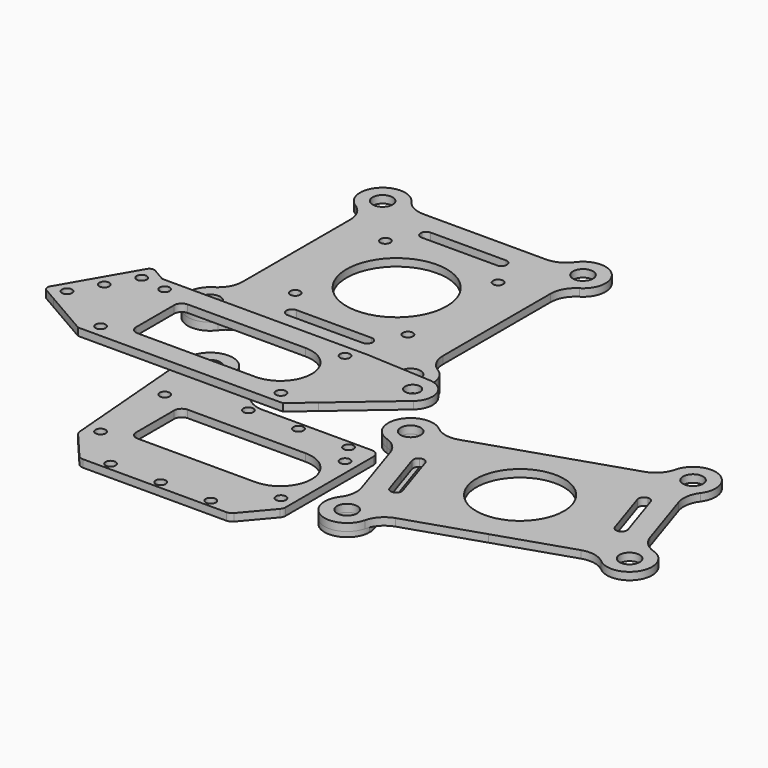
from build123d import *

# Parameters (mm, degrees)
F0_R      = 1
F0_W      = 30
F0_H      = 6.5
F0_R_2    = 2
F1_DEPTH  = 1.5
F3_R      = 2
F4_DEPTH  = 1.5
F5_R      = 5
F5_2_R    = 5
F5_3_R    = 5
F6_R      = 1.5
F7_DEPTH  = 0.5
F8_R      = 8.75
F8_R_2    = 2
F9_DEPTH  = 1.5
F10_R     = 2
F10_R_2   = 1
F10_R_3   = 10
F11_DEPTH = 1.5
F12_R     = 5
F12_2_R   = 5
F14_R     = 1
F14_R_2   = 2
F15_DEPTH = 1.5
F16_R     = 2
F17_DEPTH = 1.5
F18_R     = 1
F19_DEPTH = 1.5
F20_R     = 2
F20_R_2   = 1.5
F21_DEPTH = 1.5


with BuildPart() as f1:
    # F0 (on Top) → F1 (new body)
    with BuildSketch(Plane.XY):
        with BuildLine():
            Line((-32, -10.5), (-32, 10.5))
            Line((-32, 10.5), (9, 10.5))
            Line((9, 10.5), (9, 13.5))
            Line((9, 13.5), (-15.9210526316, 13.5))
            Line((-15.9210526316, 13.5), (-25.5, 20))
            ThreePointArc((-25.5, 20), (-29.8149179926, 15.5038077609), (-34.4847754002, 19.6301492066))
            Line((-34.4847754002, 19.6301492066), (-32, -10.5))
        make_face()
        with Locations((-16, 12)):
            Circle(F0_R, mode=Mode.SUBTRACT)
        with Locations((-6, 12)):
            Circle(F0_R, mode=Mode.SUBTRACT)
        with Locations((4, 12)):
            Circle(F0_R, mode=Mode.SUBTRACT)
        Polygon((9, 10.5), (-32, 10.5), (-32, -10.5), (-26.5, -10.5), (3.5, -10.5), (9, -10.5), align=None)
        with Locations((-29.5, -8)):
            Circle(F0_R, mode=Mode.SUBTRACT)
        with BuildLine():
            ThreePointArc((0, 6.25), (6.25, 0), (0, -6.25))
            Line((0, -6.25), (-23.5, -6.25))
            ThreePointArc((-23.5, -6.25), (-24.5606601718, -5.8106601718), (-25, -4.75))
            Line((-25, -4.75), (-25, 0))
            Line((-25, 0), (-25, 4.75))
            ThreePointArc((-25, 4.75), (-24.5606601718, 5.8106601718), (-23.5, 6.25))
            Line((-23.5, 6.25), (0, 6.25))
        make_face(mode=Mode.SUBTRACT)
        with Locations((6.5, -8)):
            Circle(F0_R, mode=Mode.SUBTRACT)
        with Locations((-29.5, 8)):
            Circle(F0_R, mode=Mode.SUBTRACT)
        with Locations((6.5, 8)):
            Circle(F0_R, mode=Mode.SUBTRACT)
        Polygon((-26.5, -10.5), (-32, -10.5), (-26.5, -17), align=None)
        Polygon((3.5, -17), (9, -10.5), (3.5, -10.5), align=None)
        with Locations((-11.5, -13.75)):
            Rectangle(F0_W, F0_H)
        with Locations((-21.5, -15.5)):
            Circle(F0_R, mode=Mode.SUBTRACT)
        with Locations((-11.5, -15.5)):
            Circle(F0_R, mode=Mode.SUBTRACT)
        with Locations((-1.5, -15.5)):
            Circle(F0_R, mode=Mode.SUBTRACT)
        with BuildLine():
            ThreePointArc((-25.5, 20), (-30.1850820074, 24.4961922391), (-34.4847754002, 19.6301492066))
            ThreePointArc((-34.4847754002, 19.6301492066), (-29.8149179926, 15.5038077609), (-25.5, 20))
        make_face()
        with Locations((-30, 20)):
            Circle(F0_R_2, mode=Mode.SUBTRACT)
    extrude(amount=F1_DEPTH)

    # F5
    f5_edges = [f1.edges().sort_by_distance(p)[0] for p in [
        (-25.5, 20, 0.75),
        (-15.921053, 13.5, 0.75),
    ]]
    fillet(f5_edges, radius=F5_R)

    # F6
    f6_edges = [f1.edges().sort_by_distance(p)[0] for p in [
        (9, -10.5, 0.75),
        (-32, -10.5, 0.75),
        (-26.5, -17, 0.75),
        (3.5, -17, 0.75),
        (9, 13.5, 0.75),
    ]]
    fillet(f6_edges, radius=F6_R)


with BuildPart() as f1b:
    # F0 (on Top) → F1, piece 2 (new body)
    with BuildSketch(Plane.XY):
        with BuildLine():
            ThreePointArc((16.9263056249, -2.74622786), (16.3601269339, -10.6255026379), (23.2938524157, -6.8404028665))
            ThreePointArc((23.2938524157, -6.8404028665), (23.2375828671, -6.1309948909), (23.0701814487, -5.4393282782))
            ThreePointArc((23.0701814487, -5.4393282782), (20.6004390973, -2.7189656704), (16.9263056249, -2.74622786))
        make_face()
        with Locations((18.7938524157, -6.8404028665)):
            Circle(F0_R_2, mode=Mode.SUBTRACT)
        with BuildLine():
            ThreePointArc((16.9263056249, -2.74622786), (20.6004390973, -2.7189656704), (23.0701814487, -5.4393282782))
            Line((23.0701814487, -5.4393282782), (14.2763290329, 21.4010745883))
            ThreePointArc((14.2763290329, 21.4010745883), (14.4437304513, 20.7094079756), (14.5, 20))
            ThreePointArc((14.5, 20), (13.4912484533, 17.1607775295), (10.9172514501, 15.5944750849))
            Line((10.9172514501, 15.5944750849), (16.9263056249, -2.74622786))
        make_face()
        with BuildLine():
            ThreePointArc((14.5, 20), (14.4437304513, 20.7094079756), (14.2763290329, 21.4010745883))
            ThreePointArc((14.2763290329, 21.4010745883), (6.1048146377, 22.2533377451), (10.9172514501, 15.5944750849))
            ThreePointArc((10.9172514501, 15.5944750849), (13.4912484533, 17.1607775295), (14.5, 20))
        make_face()
        with Locations((10, 20)):
            Circle(F0_R_2, mode=Mode.SUBTRACT)
    extrude(amount=F1_DEPTH)

    # F5#2
    f5_2_edges = [f1b.edges().sort_by_distance(p)[0] for p in [
        (10.917251, 15.594475, 0.75),
        (16.926306, -2.746228, 0.75),
    ]]
    fillet(f5_2_edges, radius=F5_2_R)

    # F7 (cut): a face of the model
    f7_faces = [f1b.faces().sort_by_distance(p)[0] for p in [
        (15.3917704428, 6.9057442473, 0),
    ]]
    extrude(f7_faces, amount=-F7_DEPTH, mode=Mode.SUBTRACT)


with BuildPart() as f4:
    # F3 (on offset) → F4 (new body)
    with BuildSketch(Plane.XY.offset(10)):
        with BuildLine():
            Line((10, 24.5), (-30, 24.5))
            ThreePointArc((-30, 24.5), (-33.3541019662, 17), (-25.527864045, 19.5))
            Line((-25.527864045, 19.5), (5.527864045, 19.5))
            ThreePointArc((5.527864045, 19.5), (13.3541019662, 17), (10, 24.5))
        make_face()
        with Locations((-30, 20)):
            Circle(F3_R, mode=Mode.SUBTRACT)
        with Locations((10, 20)):
            Circle(F3_R, mode=Mode.SUBTRACT)
    extrude(amount=F4_DEPTH)

    # F5#3
    f5_3_edges = [f4.edges().sort_by_distance(p)[0] for p in [
        (-25.527864, 19.5, 10.75),
        (5.527864, 19.5, 10.75),
    ]]
    fillet(f5_3_edges, radius=F5_3_R)


with BuildPart() as f9:
    # F8 (on face) → F9 (new body)
    with BuildSketch(Plane.XY.offset(1.5)):
        with BuildLine():
            Line((20.5635272466, 2.2114265276), (23.0701814487, -5.4393282782))
            Line((23.0701814487, -5.4393282782), (41.1257929211, 0.4763199836))
            Line((41.1257929211, 0.4763199836), (59.1814043935, 6.3919682455))
            Line((59.1814043935, 6.3919682455), (56.6747501914, 14.0427230513))
            ThreePointArc((56.6747501914, 14.0427230513), (55.7221845843, 13.9511185326), (55.0583290183, 14.6403705989))
            Line((55.0583290183, 14.6403705989), (53.5015794757, 19.3918473022))
            Line((53.5015794757, 19.3918473022), (51.9448299331, 24.1433240055))
            ThreePointArc((51.9448299331, 24.1433240055), (52.0721147828, 25.0917812742), (52.8942061798, 25.5816163062))
            Line((52.8942061798, 25.5816163062), (50.3875519777, 33.232371112))
            Line((50.3875519777, 33.232371112), (32.3319405053, 27.3167228501))
            Line((32.3319405053, 27.3167228501), (14.2763290329, 21.4010745883))
            Line((14.2763290329, 21.4010745883), (16.782983235, 13.7503197825))
            ThreePointArc((16.782983235, 13.7503197825), (17.7355488421, 13.8419243012), (18.3994044081, 13.1526722348))
            Line((18.3994044081, 13.1526722348), (19.9561539507, 8.4011955316))
            Line((19.9561539507, 8.4011955316), (21.5129034933, 3.6497188283))
            ThreePointArc((21.5129034933, 3.6497188283), (21.55382384, 3.4806447674), (21.5675786185, 3.3072339289))
            ThreePointArc((21.5675786185, 3.3072339289), (21.2786099036, 2.5641133098), (20.5635272466, 2.2114265276))
        make_face()
        with Locations((36.7288667132, 13.8965214169)):
            Circle(F8_R, mode=Mode.SUBTRACT)
        with BuildLine():
            ThreePointArc((15.175695913, -4.164782654), (18.0766255291, -11.2828780317), (23.0701814487, -5.4393282782))
            Line((23.0701814487, -5.4393282782), (20.5635272466, 2.2114265276))
            ThreePointArc((20.5635272466, 2.2114265276), (19.8616062492, 2.3891939039), (19.4222537438, 2.9647490296))
            Line((19.4222537438, 2.9647490296), (17.8655042012, 7.7162257328))
            Line((17.8655042012, 7.7162257328), (16.3087546587, 12.4677024361))
            ThreePointArc((16.3087546587, 12.4677024361), (16.3223425676, 13.1916566442), (16.782983235, 13.7503197825))
            Line((16.782983235, 13.7503197825), (14.2763290329, 21.4010745883))
            ThreePointArc((14.2763290329, 21.4010745883), (6.7929982332, 23.1567609456), (8.6666176225, 15.7020828957))
            ThreePointArc((8.6666176225, 15.7020828957), (10.6925938093, 14.489954743), (11.9365583507, 12.4833689891))
            Line((11.9365583507, 12.4833689891), (15.9069987243, 0.3648782359))
            ThreePointArc((15.9069987243, 0.3648782359), (16.0916055379, -1.9887900696), (15.175695913, -4.164782654))
        make_face()
        with Locations((18.7938524157, -6.8404028665)):
            Circle(F8_R_2, mode=Mode.SUBTRACT)
        with Locations((10, 20)):
            Circle(F8_R_2, mode=Mode.SUBTRACT)
        with BuildLine():
            Line((56.6747501914, 14.0427230513), (59.1814043935, 6.3919682455))
            ThreePointArc((59.1814043935, 6.3919682455), (66.6647351932, 4.6362818882), (64.7911158039, 12.0909599381))
            ThreePointArc((64.7911158039, 12.0909599381), (62.7651396171, 13.3030880908), (61.5211750757, 15.3096738447))
            Line((61.5211750757, 15.3096738447), (57.5507347021, 27.4281645979))
            ThreePointArc((57.5507347021, 27.4281645979), (57.3661278885, 29.7818329034), (58.2820375134, 31.9578254878))
            ThreePointArc((58.2820375134, 31.9578254878), (55.3811078973, 39.0759208655), (50.3875519777, 33.232371112))
            Line((50.3875519777, 33.232371112), (52.8942061798, 25.5816163062))
            ThreePointArc((52.8942061798, 25.5816163062), (53.5961271772, 25.4038489299), (54.0354796826, 24.8282938042))
            Line((54.0354796826, 24.8282938042), (55.5922292252, 20.076817101))
            Line((55.5922292252, 20.076817101), (57.1489787677, 15.3253403977))
            ThreePointArc((57.1489787677, 15.3253403977), (57.1898991145, 15.1562663368), (57.203653893, 14.9828554983))
            ThreePointArc((57.203653893, 14.9828554983), (57.0623524714, 14.4435067837), (56.6747501914, 14.0427230513))
        make_face()
        with Locations((63.4577334264, 7.7930428338)):
            Circle(F8_R_2, mode=Mode.SUBTRACT)
        with Locations((54.6638810107, 34.6334457003)):
            Circle(F8_R_2, mode=Mode.SUBTRACT)
    extrude(amount=F9_DEPTH)

    # F12
    f12_edges = [f9.edges().sort_by_distance(p)[0] for p in [
        (23.070181, -5.439328, 2.25),
        (59.181404, 6.391968, 2.25),
        (50.387552, 33.232371, 2.25),
        (14.276329, 21.401075, 2.25),
    ]]
    fillet(f12_edges, radius=F12_R)


with BuildPart() as f11:
    # F10 (on face) → F11 (new body)
    with BuildSketch(Plane.XY.offset(11.5)):
        with BuildLine():
            Line((-18.5712142643, 24.5), (-30, 24.5))
            ThreePointArc((-30, 24.5), (-33.9983549249, 17.9352583952), (-26.3308578825, 17.3947368421))
            ThreePointArc((-26.3308578825, 17.3947368421), (-24.5481906463, 18.9426165832), (-22.2540333076, 19.5))
            Line((-22.2540333076, 19.5), (2.2540333076, 19.5))
            ThreePointArc((2.2540333076, 19.5), (4.5481906463, 18.9426165832), (6.3308578825, 17.3947368421))
            ThreePointArc((6.3308578825, 17.3947368421), (13.9983549249, 17.9352583952), (10, 24.5))
            Line((10, 24.5), (-1.4287857357, 24.5))
            ThreePointArc((-1.4287857357, 24.5), (-1.8162602834, 23.888315603), (-2.5, 23.65))
            Line((-2.5, 23.65), (-10, 23.65))
            Line((-10, 23.65), (-17.5, 23.65))
            ThreePointArc((-17.5, 23.65), (-18.1837397166, 23.888315603), (-18.5712142643, 24.5))
        make_face()
        with Locations((-30, 20)):
            Circle(F10_R, mode=Mode.SUBTRACT)
        with Locations((10, 20)):
            Circle(F10_R, mode=Mode.SUBTRACT)
        with BuildLine():
            Line((-30, 58.5), (-30, 24.5))
            Line((-30, 24.5), (-18.5712142643, 24.5))
            ThreePointArc((-18.5712142643, 24.5), (-18.361684397, 25.4337397166), (-17.5, 25.85))
            Line((-17.5, 25.85), (-10, 25.85))
            Line((-10, 25.85), (-2.5, 25.85))
            ThreePointArc((-2.5, 25.85), (-1.7221825407, 25.5278174593), (-1.4, 24.75))
            ThreePointArc((-1.4, 24.75), (-1.4072201295, 24.6241741098), (-1.4287857357, 24.5))
            Line((-1.4287857357, 24.5), (10, 24.5))
            Line((10, 24.5), (10, 58.5))
            Line((10, 58.5), (-1.4287857357, 58.5))
            ThreePointArc((-1.4287857357, 58.5), (-1.4072201295, 58.3758258902), (-1.4, 58.25))
            ThreePointArc((-1.4, 58.25), (-1.7221825407, 57.4721825407), (-2.5, 57.15))
            Line((-2.5, 57.15), (-10, 57.15))
            Line((-10, 57.15), (-17.5, 57.15))
            ThreePointArc((-17.5, 57.15), (-18.361684397, 57.5662602834), (-18.5712142643, 58.5))
            Line((-18.5712142643, 58.5), (-30, 58.5))
        make_face()
        with Locations((-21.25, 30.25)):
            Circle(F10_R_2, mode=Mode.SUBTRACT)
        with Locations((1.25, 30.25)):
            Circle(F10_R_2, mode=Mode.SUBTRACT)
        with Locations((-10, 41.5)):
            Circle(F10_R_3, mode=Mode.SUBTRACT)
        with Locations((-21.25, 52.75)):
            Circle(F10_R_2, mode=Mode.SUBTRACT)
        with Locations((1.25, 52.75)):
            Circle(F10_R_2, mode=Mode.SUBTRACT)
        with BuildLine():
            ThreePointArc((-26.3308578825, 65.6052631579), (-33.9983549249, 65.0647416048), (-30, 58.5))
            Line((-30, 58.5), (-18.5712142643, 58.5))
            ThreePointArc((-18.5712142643, 58.5), (-18.1837397166, 59.111684397), (-17.5, 59.35))
            Line((-17.5, 59.35), (-10, 59.35))
            Line((-10, 59.35), (-2.5, 59.35))
            ThreePointArc((-2.5, 59.35), (-1.8162602834, 59.111684397), (-1.4287857357, 58.5))
            Line((-1.4287857357, 58.5), (10, 58.5))
            ThreePointArc((10, 58.5), (13.9983549249, 65.0647416048), (6.3308578825, 65.6052631579))
            ThreePointArc((6.3308578825, 65.6052631579), (4.5481906463, 64.0573834168), (2.2540333076, 63.5))
            Line((2.2540333076, 63.5), (-22.2540333076, 63.5))
            ThreePointArc((-22.2540333076, 63.5), (-24.5481906463, 64.0573834168), (-26.3308578825, 65.6052631579))
        make_face()
        with Locations((-30, 63)):
            Circle(F10_R, mode=Mode.SUBTRACT)
        with Locations((10, 63)):
            Circle(F10_R, mode=Mode.SUBTRACT)
    extrude(amount=F11_DEPTH)

    # F12#2
    f12_2_edges = [f11.edges().sort_by_distance(p)[0] for p in [
        (10, 58.5, 12.25),
        (10, 24.5, 12.25),
        (-30, 24.5, 12.25),
        (-30, 58.5, 12.25),
    ]]
    fillet(f12_2_edges, radius=F12_2_R)


with BuildPart() as f13_1:
    # F13: instance of F1
    add(f1.part.mirror(Plane.XY.offset(10)))

    # F14 (on face) → F15 (cut, through all)
    with BuildSketch(Plane.XY.offset(20)):
        with BuildLine():
            Line((-32, 10.5), (9, 10.5))
            Line((9, 10.5), (9, 12))
            ThreePointArc((9, 12), (8.5606601718, 13.0606601718), (7.5, 13.5))
            Line((7.5, 13.5), (-14.384776676, 13.5))
            ThreePointArc((-14.384776676, 13.5), (-15.8532972989, 13.7205181055), (-17.1922837676, 14.362621128))
            Line((-17.1922837676, 14.362621128), (-23.7848645846, 18.836158111))
            ThreePointArc((-23.7848645846, 18.836158111), (-24.9684160432, 19.9616519173), (-25.7261167072, 21.4085175182))
            ThreePointArc((-25.7261167072, 21.4085175182), (-30.8954146153, 24.4100150416), (-34.4847754002, 19.6301492066))
            Line((-34.4847754002, 19.6301492066), (-32.0394894317, -10.0211549227))
            ThreePointArc((-32.0394894317, -10.0211549227), (-32.0246024748, -10.1417708861), (-32, -10.2607858026))
            Line((-32, -10.2607858026), (-32, 10.5))
        make_face()
        with Locations((-16, 12)):
            Circle(F14_R, mode=Mode.SUBTRACT)
        with Locations((-30, 20)):
            Circle(F14_R_2, mode=Mode.SUBTRACT)
        with Locations((-6, 12)):
            Circle(F14_R, mode=Mode.SUBTRACT)
        with Locations((4, 12)):
            Circle(F14_R, mode=Mode.SUBTRACT)
        with BuildLine():
            ThreePointArc((8.6450794281, -10.919451585), (8.7876049399, -10.7200013595), (8.895740576, -10.5))
            Line((8.895740576, -10.5), (-31.9184060135, -10.5))
            ThreePointArc((-31.9184060135, -10.5), (-31.8173068815, -10.6916762863), (-31.6896437263, -10.8667846871))
            Line((-31.6896437263, -10.8667846871), (-26.9493810012, -16.4689133622))
            ThreePointArc((-26.9493810012, -16.4689133622), (-26.4354235727, -16.8607663362), (-25.8043015732, -17))
            Line((-25.8043015732, -17), (2.8043015732, -17))
            ThreePointArc((2.8043015732, -17), (3.4354235727, -16.8607663362), (3.9493810012, -16.4689133622))
            Line((3.9493810012, -16.4689133622), (8.6450794281, -10.919451585))
        make_face()
        with Locations((-21.5, -15.5)):
            Circle(F14_R, mode=Mode.SUBTRACT)
        with Locations((-11.5, -15.5)):
            Circle(F14_R, mode=Mode.SUBTRACT)
        with Locations((-1.5, -15.5)):
            Circle(F14_R, mode=Mode.SUBTRACT)
    extrude(amount=-F15_DEPTH, mode=Mode.SUBTRACT)

    # F16 (on face) + F14 (on face) → F17 (join)
    with BuildSketch(Plane.XY.offset(20)):
        with BuildLine():
            Line((13.0820683905, -6.8977674396), (24.3423168571, 2.7914006002))
            ThreePointArc((24.3423168571, 2.7914006002), (25.5188626027, 7.1156170374), (21.9438310361, 9.8178858964))
            Line((21.9438310361, 9.8178858964), (9, 10.5))
            Line((9, 10.5), (9, 0.2747308886))
            Line((9, 0.2747308886), (13.0820683905, -6.8977674396))
        make_face()
        with Locations((21.7333310915, 5.8234285148)):
            Circle(F16_R, mode=Mode.SUBTRACT)
        with BuildLine():
            Line((8.895740576, -10.5), (13.0820683905, -6.8977674396))
            Line((13.0820683905, -6.8977674396), (9, 0.2747308886))
            Line((9, 0.2747308886), (9, -9.9505382228))
            ThreePointArc((9, -9.9505382228), (8.9737046624, -10.2301711394), (8.895740576, -10.5))
        make_face()
    with BuildSketch(Plane.XY.offset(20)):
        with BuildLine():
            ThreePointArc((-31.9184060135, -10.5), (-31.964250367, -10.3821145142), (-32, -10.2607858026))
            Line((-32, -10.2607858026), (-32, -10.5))
            Line((-32, -10.5), (-31.9184060135, -10.5))
        make_face()
    extrude(amount=-F17_DEPTH)

    # F18 (on face) → F19 (join)
    with BuildSketch(Plane.XY.offset(20)):
        Polygon((-41.0932667397, -5.25), (-32, -10.5), (-32, 10.5), align=None)
        Polygon((-43.6913429511, -3.75), (-41.0932667397, -5.25), (-32, 10.5), (-34.5980762114, 12), align=None)
        with Locations((-40.9706714755, -2.0376587737)):
            Circle(F18_R, mode=Mode.SUBTRACT)
        with Locations((-37.8456714755, 3.375)):
            Circle(F18_R, mode=Mode.SUBTRACT)
        with Locations((-34.7206714755, 8.7876587737)):
            Circle(F18_R, mode=Mode.SUBTRACT)
        with BuildLine():
            ThreePointArc((-44.0573683549, -2.3839745962), (-44.1572687774, -3.1427936413), (-43.6913429511, -3.75))
            Line((-43.6913429511, -3.75), (-34.5980762114, 12))
            ThreePointArc((-34.5980762114, 12), (-35.3568952565, 12.0999004225), (-35.9641016151, 11.6339745962))
            Line((-35.9641016151, 11.6339745962), (-44.0573683549, -2.3839745962))
        make_face()
    extrude(amount=-F19_DEPTH)

    # F20 (on face) → F21 (join)
    with BuildSketch(Plane.XY.offset(20)):
        with Locations((21.7333310915, 5.8234285148)):
            Circle(F20_R)
        with Locations((21.7333310915, 5.8234285148)):
            Circle(F20_R_2, mode=Mode.SUBTRACT)
    extrude(amount=-F21_DEPTH)


solid = Compound([f1.part, f1b.part, f4.part, f9.part, f11.part, f13_1.part])
